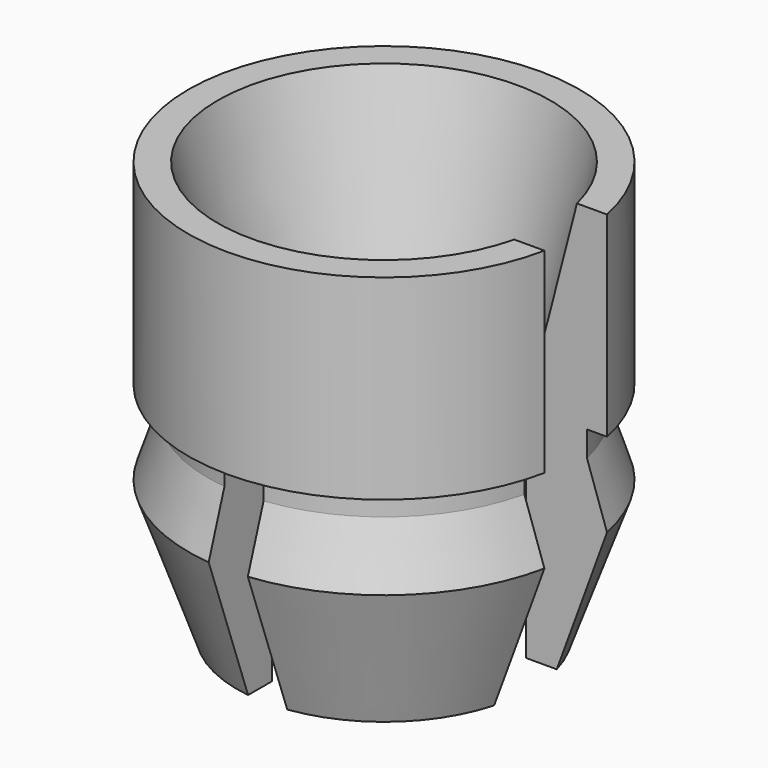
from build123d import *

# Parameters (mm, degrees)
F6_R       = 7.5
F3_R       = 10
F0_R       = 9
F7_FACE_R  = 10
F9_DEPTH   = 1.3
F11_R      = 10
F11_R_2    = 9
F12_DEPTH  = 10
F10_R      = 6
F14_DEPTH  = 11.3
F15_R      = 8.5
F14_FACE_R = 6
F13_W      = 2
F13_H      = 2
F17_DEPTH  = 11.3
F18_DEPTH  = 21.3010001


with BuildPart() as f7:
    # F6 (on plane+point) → F7 section 0
    with BuildSketch(Plane.XY.offset(-10)):
        Circle(F6_R)
    # F3 (on plane+point) → F7 section 1
    with BuildSketch(Plane.XY.offset(-3)):
        Circle(F3_R)
    loft()

    # F0 (on Top) → F8 section 0
    with BuildSketch(Plane.XY):
        Circle(F0_R)
    # F7_face (on face) → F8 section 1
    with BuildSketch(Plane.XY.offset(-3)):
        Circle(F7_FACE_R)
    loft()

    # F9 (add): a face of the model
    f9_faces = [f7.faces().sort_by_distance(p)[0] for p in [
        (0, 0, 0),
    ]]
    extrude(f9_faces, amount=F9_DEPTH)

    # F11 (on face) → F12 (join)
    with BuildSketch(Plane.XY.offset(1.3)):
        Circle(F11_R)
        Circle(F11_R_2, mode=Mode.SUBTRACT)
        Circle(F11_R_2)
    extrude(amount=F12_DEPTH)

    # F10 (on face) → F14 (cut, through all)
    with BuildSketch(Plane(origin=(0, 0, -10), x_dir=(1, 0, 0), z_dir=(0, 0, -1))):
        Circle(F10_R)
    extrude(amount=-F14_DEPTH, mode=Mode.SUBTRACT)

    # F15 (on face) → F16 section 0
    with BuildSketch(Plane.XY.offset(11.3)):
        Circle(F15_R)
    # F14_face (on face) → F16 section 1
    with BuildSketch(Plane(origin=(0, 0, 1.3), x_dir=(1, 0, 0), z_dir=(0, 0, -1))):
        Circle(F14_FACE_R)
    loft(mode=Mode.SUBTRACT)

    # F13 (on face) → F17 (cut, through all)
    with BuildSketch(Plane(origin=(0, 0, -10), x_dir=(1, 0, 0), z_dir=(0, 0, -1))):
        with BuildLine():
            Line((-1, 15), (-1, 7.4330343737))
            ThreePointArc((-1, 7.4330343737), (0, 7.5), (1, 7.4330343737))
            Line((1, 7.4330343737), (1, 15))
            Line((1, 15), (-1, 15))
        make_face()
        with BuildLine():
            Line((-1, 7.4330343737), (-1, 1))
            Line((-1, 1), (1, 1))
            Line((1, 1), (1, 2))
            Line((1, 2), (1, 7.4330343737))
            ThreePointArc((1, 7.4330343737), (0, 7.5), (-1, 7.4330343737))
        make_face()
        with BuildLine():
            Line((15, 1), (7.4330343737, 1))
            ThreePointArc((7.4330343737, 1), (7.4832398666, 0.5011198447), (7.5, 0))
            ThreePointArc((7.5, 0), (7.4832398666, -0.5011198447), (7.4330343737, -1))
            Line((7.4330343737, -1), (15, -1))
            Line((15, -1), (15, 1))
        make_face()
        with BuildLine():
            Line((7.4330343737, 1), (1, 1))
            Line((1, 1), (1, -1))
            Line((1, -1), (7.4330343737, -1))
            ThreePointArc((7.4330343737, -1), (7.4832398666, -0.5011198447), (7.5, 0))
            ThreePointArc((7.5, 0), (7.4832398666, 0.5011198447), (7.4330343737, 1))
        make_face()
        with BuildLine():
            Line((-7.4330343737, 1), (-15, 1))
            Line((-15, 1), (-15, -1))
            Line((-15, -1), (-7.4330343737, -1))
            ThreePointArc((-7.4330343737, -1), (-7.5, 0), (-7.4330343737, 1))
        make_face()
        with BuildLine():
            Line((-1, 1), (-7.4330343737, 1))
            ThreePointArc((-7.4330343737, 1), (-7.5, 0), (-7.4330343737, -1))
            Line((-7.4330343737, -1), (-1, -1))
            Line((-1, -1), (-1, 1))
        make_face()
        Rectangle(F13_W, F13_H)
        with BuildLine():
            Line((1, -1), (-1, -1))
            Line((-1, -1), (-1, -7.4330343737))
            ThreePointArc((-1, -7.4330343737), (0, -7.5), (1, -7.4330343737))
            Line((1, -7.4330343737), (1, -2))
            Line((1, -2), (1, -1))
        make_face()
        with BuildLine():
            ThreePointArc((1, -7.4330343737), (0, -7.5), (-1, -7.4330343737))
            Line((-1, -7.4330343737), (-1, -15))
            Line((-1, -15), (1, -15))
            Line((1, -15), (1, -7.4330343737))
        make_face()
    extrude(amount=-F17_DEPTH, mode=Mode.SUBTRACT)

    # F13 (on face) → F18 (cut, through all)
    with BuildSketch(Plane(origin=(0, 0, -10), x_dir=(1, 0, 0), z_dir=(0, 0, -1))):
        with BuildLine():
            Line((7.4330343737, -1), (1, -1))
            Line((1, -1), (1, -2))
            Line((1, -2), (7.2284161474, -2))
            ThreePointArc((7.2284161474, -2), (7.3477569942, -1.5034850031), (7.4330343737, -1))
        make_face()
        with BuildLine():
            Line((7.4330343737, 1), (1, 1))
            Line((1, 1), (1, -1))
            Line((1, -1), (7.4330343737, -1))
            ThreePointArc((7.4330343737, -1), (7.4832398666, -0.5011198447), (7.5, 0))
            ThreePointArc((7.5, 0), (7.4832398666, 0.5011198447), (7.4330343737, 1))
        make_face()
        with BuildLine():
            Line((1, 2), (1, 1))
            Line((1, 1), (7.4330343737, 1))
            ThreePointArc((7.4330343737, 1), (7.3477569942, 1.5034850031), (7.2284161474, 2))
            Line((7.2284161474, 2), (1, 2))
        make_face()
        with BuildLine():
            ThreePointArc((7.2284161474, 2), (7.3477569942, 1.5034850031), (7.4330343737, 1))
            Line((7.4330343737, 1), (15, 1))
            Line((15, 1), (15, 2))
            Line((15, 2), (7.2284161474, 2))
        make_face()
        with BuildLine():
            Line((15, 1), (7.4330343737, 1))
            ThreePointArc((7.4330343737, 1), (7.4832398666, 0.5011198447), (7.5, 0))
            ThreePointArc((7.5, 0), (7.4832398666, -0.5011198447), (7.4330343737, -1))
            Line((7.4330343737, -1), (15, -1))
            Line((15, -1), (15, 1))
        make_face()
        with BuildLine():
            Line((15, -1), (7.4330343737, -1))
            ThreePointArc((7.4330343737, -1), (7.3477569942, -1.5034850031), (7.2284161474, -2))
            Line((7.2284161474, -2), (15, -2))
            Line((15, -2), (15, -1))
        make_face()
    extrude(amount=-F18_DEPTH, mode=Mode.SUBTRACT)


solid = f7.part
